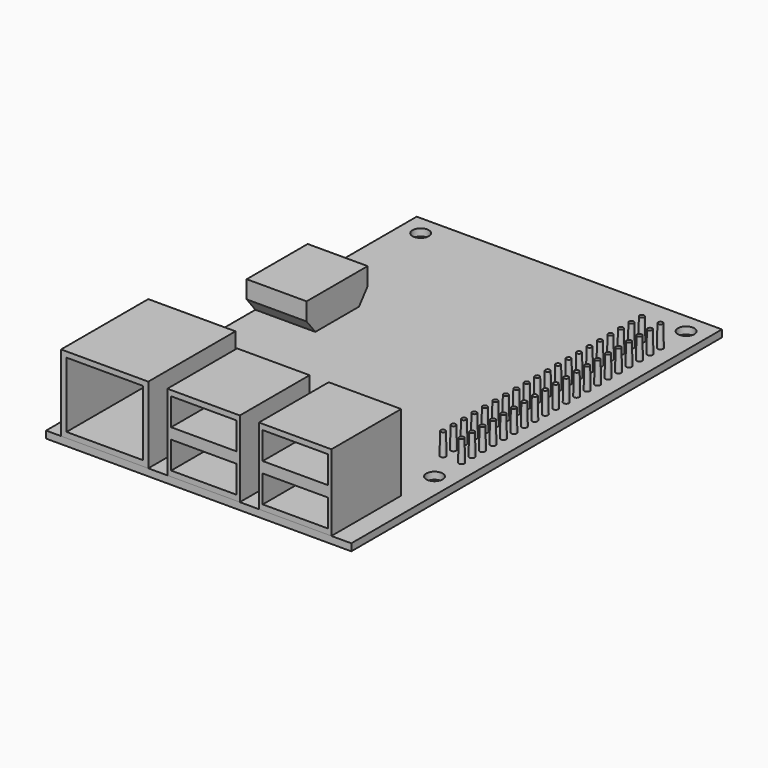
from build123d import *

# Parameters (mm, degrees)
F0_W      = 56
F0_H      = 85
F0_R      = 1.5
F1_DEPTH  = 1.3
F2_W      = 16
F2_H      = 20
F3_DEPTH  = 14
F2_W_2    = 13.3
F2_H_2    = 16
F4_T      = -1
F5_W      = 12
F5_H      = 5
F6_DEPTH  = 15
F8_DEPTH  = 11
F9_T      = -1
F10_R     = 0.5
F11_DEPTH = 4
F11_TAPER = 1


with BuildPart() as f1:
    # F0 (on Top) → F1 (new body)
    with BuildSketch(Plane.XY):
        Rectangle(F0_W, F0_H)
        with Locations((-24.35, -18.85)):
            Circle(F0_R, mode=Mode.SUBTRACT)
        with Locations((24.35, -18.85)):
            Circle(F0_R, mode=Mode.SUBTRACT)
        with Locations((-24.35, 38.85)):
            Circle(F0_R, mode=Mode.SUBTRACT)
        with Locations((24.35, 38.85)):
            Circle(F0_R, mode=Mode.SUBTRACT)
    extrude(amount=F1_DEPTH)


with BuildPart() as f3:
    # F2 (on face) → F3 (new body)
    with BuildSketch(Plane.XY.offset(1.3)):
        with Locations((-17.25, -32.5)):
            Rectangle(F2_W, F2_H)
    extrude(amount=F3_DEPTH)

    # F4
    f4_openings = [f3.faces().sort_by_distance(p)[0] for p in [
        (-17.25, -42.5, 8.3),
    ]]
    offset(amount=F4_T, openings=f4_openings)


with BuildPart() as f3b:
    # F2 (on face) → F3, piece 2 (new body)
    with BuildSketch(Plane.XY.offset(1.3)):
        with Locations((0.9, -34.5)):
            Rectangle(F2_W_2, F2_H_2)
    extrude(amount=F3_DEPTH)


with BuildPart() as f3c:
    # F2 (on face) → F3, piece 3 (new body)
    with BuildSketch(Plane.XY.offset(1.3)):
        with Locations((17.7, -34.5)):
            Rectangle(F2_W_2, F2_H_2)
    extrude(amount=F3_DEPTH)


with BuildPart() as f6_tool:
    # F5 (on face) → F6 (new body, through all)
    with BuildSketch(Plane.XZ.offset(42.5)):
        with Locations((0.95, 11.8)):
            Rectangle(F5_W, F5_H)
        with Locations((0.95, 4.8)):
            Rectangle(F5_W, F5_H)
        with Locations((17.75, 11.8)):
            Rectangle(F5_W, F5_H)
        with Locations((17.75, 4.8)):
            Rectangle(F5_W, F5_H)
    extrude(amount=-F6_DEPTH)


with BuildPart() as f3b_1:
    add(f3b.part)

    # F6: cut by f6_tool
    add(f6_tool.part, mode=Mode.SUBTRACT)


with BuildPart() as f3c_1:
    add(f3c.part)

    # F6: cut by f6_tool
    add(f6_tool.part, mode=Mode.SUBTRACT)


with BuildPart() as f8:
    # F7 (on face) → F8 (new body)
    with BuildSketch(Plane(origin=(-28, 0, 0), x_dir=(0, -1, 0), z_dir=(-1, 0, 0))):
        Polygon((-17.5, 3.7962250415), (-15.5, 1.3), (-5.5, 1.3), (-3.5, 3.7962250415), (-3.5, 7.05), (-17.5, 7.05), align=None)
    extrude(amount=-F8_DEPTH)

    # F9
    f9_openings = [f8.faces().sort_by_distance(p)[0] for p in [
        (-28, 10.5, 4.310075),
    ]]
    offset(amount=F9_T, openings=f9_openings)


with BuildPart() as f11:
    # F10 (on face) → F11 (new body)
    with BuildSketch(Plane.XY.offset(1.3)):
        with Locations((21.292258054, 32.522983849)):
            Circle(F10_R)
    extrude(amount=F11_DEPTH, taper=F11_TAPER)


with BuildPart() as f11b:
    # F10 (on face) → F11, piece 2 (new body)
    with BuildSketch(Plane.XY.offset(1.3)):
        with Locations((21.292258054, 30.122983849)):
            Circle(F10_R)
    extrude(amount=F11_DEPTH, taper=F11_TAPER)


with BuildPart() as f11c:
    # F10 (on face) → F11, piece 3 (new body)
    with BuildSketch(Plane.XY.offset(1.3)):
        with Locations((21.292258054, 27.722983849)):
            Circle(F10_R)
    extrude(amount=F11_DEPTH, taper=F11_TAPER)


with BuildPart() as f11d:
    # F10 (on face) → F11, piece 4 (new body)
    with BuildSketch(Plane.XY.offset(1.3)):
        with Locations((21.292258054, 25.322983849)):
            Circle(F10_R)
    extrude(amount=F11_DEPTH, taper=F11_TAPER)


with BuildPart() as f11e:
    # F10 (on face) → F11, piece 5 (new body)
    with BuildSketch(Plane.XY.offset(1.3)):
        with Locations((21.292258054, 22.922983849)):
            Circle(F10_R)
    extrude(amount=F11_DEPTH, taper=F11_TAPER)


with BuildPart() as f11f:
    # F10 (on face) → F11, piece 6 (new body)
    with BuildSketch(Plane.XY.offset(1.3)):
        with Locations((21.292258054, 20.522983849)):
            Circle(F10_R)
    extrude(amount=F11_DEPTH, taper=F11_TAPER)


with BuildPart() as f11g:
    # F10 (on face) → F11, piece 7 (new body)
    with BuildSketch(Plane.XY.offset(1.3)):
        with Locations((21.292258054, 18.122983849)):
            Circle(F10_R)
    extrude(amount=F11_DEPTH, taper=F11_TAPER)


with BuildPart() as f11h:
    # F10 (on face) → F11, piece 8 (new body)
    with BuildSketch(Plane.XY.offset(1.3)):
        with Locations((21.292258054, 15.722983849)):
            Circle(F10_R)
    extrude(amount=F11_DEPTH, taper=F11_TAPER)


with BuildPart() as f11i:
    # F10 (on face) → F11, piece 9 (new body)
    with BuildSketch(Plane.XY.offset(1.3)):
        with Locations((21.292258054, 13.322983849)):
            Circle(F10_R)
    extrude(amount=F11_DEPTH, taper=F11_TAPER)


with BuildPart() as f11j:
    # F10 (on face) → F11, piece 10 (new body)
    with BuildSketch(Plane.XY.offset(1.3)):
        with Locations((21.292258054, 10.922983849)):
            Circle(F10_R)
    extrude(amount=F11_DEPTH, taper=F11_TAPER)


with BuildPart() as f11k:
    # F10 (on face) → F11, piece 11 (new body)
    with BuildSketch(Plane.XY.offset(1.3)):
        with Locations((21.292258054, 8.522983849)):
            Circle(F10_R)
    extrude(amount=F11_DEPTH, taper=F11_TAPER)


with BuildPart() as f11l:
    # F10 (on face) → F11, piece 12 (new body)
    with BuildSketch(Plane.XY.offset(1.3)):
        with Locations((21.292258054, 6.122983849)):
            Circle(F10_R)
    extrude(amount=F11_DEPTH, taper=F11_TAPER)


with BuildPart() as f11m:
    # F10 (on face) → F11, piece 13 (new body)
    with BuildSketch(Plane.XY.offset(1.3)):
        with Locations((21.292258054, 3.722983849)):
            Circle(F10_R)
    extrude(amount=F11_DEPTH, taper=F11_TAPER)


with BuildPart() as f11n:
    # F10 (on face) → F11, piece 14 (new body)
    with BuildSketch(Plane.XY.offset(1.3)):
        with Locations((21.292258054, 1.322983849)):
            Circle(F10_R)
    extrude(amount=F11_DEPTH, taper=F11_TAPER)


with BuildPart() as f11o:
    # F10 (on face) → F11, piece 15 (new body)
    with BuildSketch(Plane.XY.offset(1.3)):
        with Locations((21.292258054, -1.077016151)):
            Circle(F10_R)
    extrude(amount=F11_DEPTH, taper=F11_TAPER)


with BuildPart() as f11p:
    # F10 (on face) → F11, piece 16 (new body)
    with BuildSketch(Plane.XY.offset(1.3)):
        with Locations((21.292258054, -3.477016151)):
            Circle(F10_R)
    extrude(amount=F11_DEPTH, taper=F11_TAPER)


with BuildPart() as f11q:
    # F10 (on face) → F11, piece 17 (new body)
    with BuildSketch(Plane.XY.offset(1.3)):
        with Locations((21.292258054, -5.877016151)):
            Circle(F10_R)
    extrude(amount=F11_DEPTH, taper=F11_TAPER)


with BuildPart() as f11r:
    # F10 (on face) → F11, piece 18 (new body)
    with BuildSketch(Plane.XY.offset(1.3)):
        with Locations((21.292258054, -8.277016151)):
            Circle(F10_R)
    extrude(amount=F11_DEPTH, taper=F11_TAPER)


with BuildPart() as f11s:
    # F10 (on face) → F11, piece 19 (new body)
    with BuildSketch(Plane.XY.offset(1.3)):
        with Locations((21.292258054, -10.677016151)):
            Circle(F10_R)
    extrude(amount=F11_DEPTH, taper=F11_TAPER)


with BuildPart() as f11t:
    # F10 (on face) → F11, piece 20 (new body)
    with BuildSketch(Plane.XY.offset(1.3)):
        with Locations((21.292258054, -13.077016151)):
            Circle(F10_R)
    extrude(amount=F11_DEPTH, taper=F11_TAPER)


with BuildPart() as f11u:
    # F10 (on face) → F11, piece 21 (new body)
    with BuildSketch(Plane.XY.offset(1.3)):
        with Locations((24.692258054, 32.522983849)):
            Circle(F10_R)
    extrude(amount=F11_DEPTH, taper=F11_TAPER)


with BuildPart() as f11v:
    # F10 (on face) → F11, piece 22 (new body)
    with BuildSketch(Plane.XY.offset(1.3)):
        with Locations((24.692258054, 30.122983849)):
            Circle(F10_R)
    extrude(amount=F11_DEPTH, taper=F11_TAPER)


with BuildPart() as f11w:
    # F10 (on face) → F11, piece 23 (new body)
    with BuildSketch(Plane.XY.offset(1.3)):
        with Locations((24.692258054, 27.722983849)):
            Circle(F10_R)
    extrude(amount=F11_DEPTH, taper=F11_TAPER)


with BuildPart() as f11x:
    # F10 (on face) → F11, piece 24 (new body)
    with BuildSketch(Plane.XY.offset(1.3)):
        with Locations((24.692258054, 25.322983849)):
            Circle(F10_R)
    extrude(amount=F11_DEPTH, taper=F11_TAPER)


with BuildPart() as f11y:
    # F10 (on face) → F11, piece 25 (new body)
    with BuildSketch(Plane.XY.offset(1.3)):
        with Locations((24.692258054, 22.922983849)):
            Circle(F10_R)
    extrude(amount=F11_DEPTH, taper=F11_TAPER)


with BuildPart() as f11z:
    # F10 (on face) → F11, piece 26 (new body)
    with BuildSketch(Plane.XY.offset(1.3)):
        with Locations((24.692258054, 20.522983849)):
            Circle(F10_R)
    extrude(amount=F11_DEPTH, taper=F11_TAPER)


with BuildPart() as f11ba:
    # F10 (on face) → F11, piece 27 (new body)
    with BuildSketch(Plane.XY.offset(1.3)):
        with Locations((24.692258054, 18.122983849)):
            Circle(F10_R)
    extrude(amount=F11_DEPTH, taper=F11_TAPER)


with BuildPart() as f11bb:
    # F10 (on face) → F11, piece 28 (new body)
    with BuildSketch(Plane.XY.offset(1.3)):
        with Locations((24.692258054, 15.722983849)):
            Circle(F10_R)
    extrude(amount=F11_DEPTH, taper=F11_TAPER)


with BuildPart() as f11bc:
    # F10 (on face) → F11, piece 29 (new body)
    with BuildSketch(Plane.XY.offset(1.3)):
        with Locations((24.692258054, 13.322983849)):
            Circle(F10_R)
    extrude(amount=F11_DEPTH, taper=F11_TAPER)


with BuildPart() as f11bd:
    # F10 (on face) → F11, piece 30 (new body)
    with BuildSketch(Plane.XY.offset(1.3)):
        with Locations((24.692258054, 10.922983849)):
            Circle(F10_R)
    extrude(amount=F11_DEPTH, taper=F11_TAPER)


with BuildPart() as f11be:
    # F10 (on face) → F11, piece 31 (new body)
    with BuildSketch(Plane.XY.offset(1.3)):
        with Locations((24.692258054, 8.522983849)):
            Circle(F10_R)
    extrude(amount=F11_DEPTH, taper=F11_TAPER)


with BuildPart() as f11bf:
    # F10 (on face) → F11, piece 32 (new body)
    with BuildSketch(Plane.XY.offset(1.3)):
        with Locations((24.692258054, 6.122983849)):
            Circle(F10_R)
    extrude(amount=F11_DEPTH, taper=F11_TAPER)


with BuildPart() as f11bg:
    # F10 (on face) → F11, piece 33 (new body)
    with BuildSketch(Plane.XY.offset(1.3)):
        with Locations((24.692258054, 3.722983849)):
            Circle(F10_R)
    extrude(amount=F11_DEPTH, taper=F11_TAPER)


with BuildPart() as f11bh:
    # F10 (on face) → F11, piece 34 (new body)
    with BuildSketch(Plane.XY.offset(1.3)):
        with Locations((24.692258054, 1.322983849)):
            Circle(F10_R)
    extrude(amount=F11_DEPTH, taper=F11_TAPER)


with BuildPart() as f11bi:
    # F10 (on face) → F11, piece 35 (new body)
    with BuildSketch(Plane.XY.offset(1.3)):
        with Locations((24.692258054, -1.077016151)):
            Circle(F10_R)
    extrude(amount=F11_DEPTH, taper=F11_TAPER)


with BuildPart() as f11bj:
    # F10 (on face) → F11, piece 36 (new body)
    with BuildSketch(Plane.XY.offset(1.3)):
        with Locations((24.692258054, -3.477016151)):
            Circle(F10_R)
    extrude(amount=F11_DEPTH, taper=F11_TAPER)


with BuildPart() as f11bk:
    # F10 (on face) → F11, piece 37 (new body)
    with BuildSketch(Plane.XY.offset(1.3)):
        with Locations((24.692258054, -5.877016151)):
            Circle(F10_R)
    extrude(amount=F11_DEPTH, taper=F11_TAPER)


with BuildPart() as f11bl:
    # F10 (on face) → F11, piece 38 (new body)
    with BuildSketch(Plane.XY.offset(1.3)):
        with Locations((24.692258054, -8.277016151)):
            Circle(F10_R)
    extrude(amount=F11_DEPTH, taper=F11_TAPER)


with BuildPart() as f11bm:
    # F10 (on face) → F11, piece 39 (new body)
    with BuildSketch(Plane.XY.offset(1.3)):
        with Locations((24.692258054, -10.677016151)):
            Circle(F10_R)
    extrude(amount=F11_DEPTH, taper=F11_TAPER)


with BuildPart() as f11bn:
    # F10 (on face) → F11, piece 40 (new body)
    with BuildSketch(Plane.XY.offset(1.3)):
        with Locations((24.692258054, -13.077016151)):
            Circle(F10_R)
    extrude(amount=F11_DEPTH, taper=F11_TAPER)


solid = Compound([f1.part, f3.part, f3b_1.part, f3c_1.part, f8.part, f11.part, f11b.part, f11c.part, f11d.part, f11e.part, f11f.part, f11g.part, f11h.part, f11i.part, f11j.part, f11k.part, f11l.part, f11m.part, f11n.part, f11o.part, f11p.part, f11q.part, f11r.part, f11s.part, f11t.part, f11u.part, f11v.part, f11w.part, f11x.part, f11y.part, f11z.part, f11ba.part, f11bb.part, f11bc.part, f11bd.part, f11be.part, f11bf.part, f11bg.part, f11bh.part, f11bi.part, f11bj.part, f11bk.part, f11bl.part, f11bm.part, f11bn.part])
